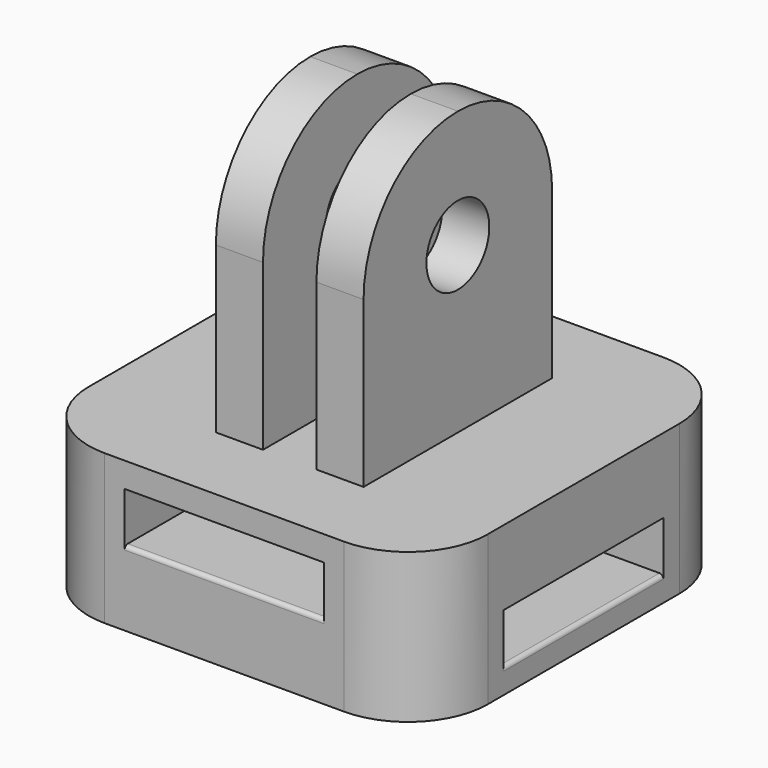
from build123d import *

# Parameters (mm, degrees)
F0_W     = 25.4
F0_H     = 25.4
F1_DEPTH = 9.525
F2_W     = 3
F2_H     = 15
F3_DEPTH = 18
F4_R     = 7.49999
F5_W     = 12.7
F5_H     = 3.175
F6_DEPTH = 25.401
F7_W     = 12.7
F7_H     = 3.175
F8_DEPTH = 25.401
F10_D    = 5
F11_R    = 5.08
F12_R    = 0.254


# Not quite as in the source:
# - a fillet or chamfer is up to 0.001 mm smaller than in the source, because OpenCascade refuses the exact size


with BuildPart() as f1:
    # F0 (on Top) → F1 (new body)
    with BuildSketch(Plane.XY):
        Rectangle(F0_W, F0_H)
    extrude(amount=F1_DEPTH)

    # F2 (on face) → F3 (join)
    with BuildSketch(Plane.XY.offset(9.525)):
        with Locations((-3.2, 0)):
            Rectangle(F2_W, F2_H)
        with Locations((3.2, 0)):
            Rectangle(F2_W, F2_H)
    extrude(amount=F3_DEPTH)

    # F4 (radius 7.5 in the source; OpenCascade refuses exactly that, so slightly less here)
    f4_edges = [f1.edges().sort_by_distance(p)[0] for p in [
        (3.2, 7.5, 27.525),
        (3.2, -7.5, 27.525),
        (-3.2, 7.5, 27.525),
        (-3.2, -7.5, 27.525),
    ]]
    fillet(f4_edges, radius=F4_R)

    # F5 (on face) → F6 (cut, through all)
    with BuildSketch(Plane.YZ.offset(12.7)):
        with Locations((0, 3.175)):
            Rectangle(F5_W, F5_H)
    extrude(amount=-F6_DEPTH, mode=Mode.SUBTRACT)

    # F7 (on face) → F8 (cut, through all)
    with BuildSketch(Plane.XZ.offset(12.7)):
        with Locations((0, 6.35)):
            Rectangle(F7_W, F7_H)
    extrude(amount=-F8_DEPTH, mode=Mode.SUBTRACT)

    # F10 (through all)
    with Locations(Plane.YZ.offset(4.7)):
        with Locations((0, 20.025)):
            Hole(F10_D / 2)

    # F11
    f11_edges = [f1.edges().sort_by_distance(p)[0] for p in [
        (12.7, -12.7, 4.7625),
        (-12.7, -12.7, 4.7625),
        (12.7, 12.7, 4.7625),
        (-12.7, 12.7, 4.7625),
    ]]
    fillet(f11_edges, radius=F11_R)

    # F12
    f12_edges = [f1.edges().sort_by_distance(p)[0] for p in [
        (0, -12.7, 4.7625),
        (12.7, 0, 1.5875),
        (0, 12.7, 4.7625),
        (-12.7, 0, 1.5875),
    ]]
    fillet(f12_edges, radius=F12_R)


solid = f1.part
